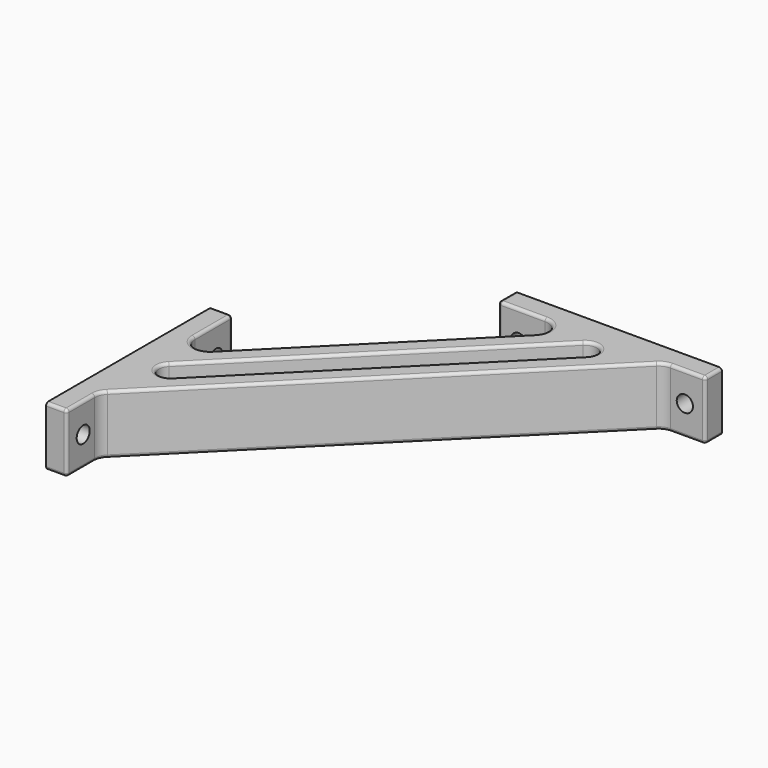
from build123d import *

# Parameters (mm, degrees)
F1_DEPTH       = 20
F6_D           = 5.5
F6_DEPTH       = 7.001
F6_ON_F3_D     = 5.5
F6_ON_F4_D     = 5.5
F6_ON_F4_DEPTH = 7.001
F6_ON_F2_D     = 5.5
F7_R           = 5
F8_R           = 5
F10_DEPTH      = 20.001
F11_R          = 1


# Not quite as in the source:
# - a feature names something its author has since deleted; it is built from what else it names


with BuildPart() as f1:
    # F0 (on Top) → F1 (new body)
    with BuildSketch(Plane.XY):
        Polygon((71.2901826474, 58.548764092), (43.0059113999, 58.548764092), (-34.7758345306, -19.2329818385), (-34.7758345306, -47.517253086), align=None)
        Polygon((85.1480470237, 65.548764092), (15.1480470237, 65.548764092), (15.1480470237, 58.548764092), (43.0059113999, 58.548764092), (71.2901826474, 58.548764092), (85.1480470237, 58.548764092), align=None)
        Polygon((-34.7758345306, -47.517253086), (-34.7758345306, -19.2329818385), (-34.7758345306, 8.6248825378), (-41.7758345306, 8.6248825378), (-41.7758345306, -61.3751174622), (-34.7758345306, -61.3751174622), align=None)
    extrude(amount=-F1_DEPTH)

    # F6 (through all, one way)
    with BuildSketch(Plane.YZ.offset(-34.7758345306)):
        with Locations((1.6958825378, -10)):
            Circle(F6_D / 2)
    extrude(amount=-F6_DEPTH, mode=Mode.SUBTRACT)

    # F6 on F3 (through all)
    with Locations(Plane.YZ.offset(-34.7758345306)):
        with Locations((-54.4461852741, -10)):
            Hole(F6_ON_F3_D / 2)

    # F6 on F4 (through all, one way)
    with BuildSketch(Plane.XZ.offset(-58.548764092)):
        with Locations((22.0770470237, -10)):
            Circle(F6_ON_F4_D / 2)
    extrude(amount=-F6_ON_F4_DEPTH, mode=Mode.SUBTRACT)

    # F6 on F2 (through all)
    with Locations(Plane.XZ.offset(-58.548764092)):
        with Locations((78.2191148355, -10)):
            Hole(F6_ON_F2_D / 2)

    # F7
    f7_edges = [f1.edges().sort_by_distance(p)[0] for p in [
        (-34.775835, -47.517253, -10),
        (71.290183, 58.548764, -10),
    ]]
    fillet(f7_edges, radius=F7_R)

    # F8
    f8_edges = [f1.edges().sort_by_distance(p)[0] for p in [
        (-34.775835, -19.232982, -10),
        (43.005911, 58.548764, -10),
    ]]
    fillet(f8_edges, radius=F8_R)

    # F9 (on face) → F10 (cut, through all)
    with BuildSketch(Plane(origin=(0, 0, -20), x_dir=(1, 0, 0), z_dir=(0, 0, -1))):
        with BuildLine():
            ThreePointArc((47.248552087, -54.3061234049), (52.9054063365, -54.3061234049), (52.9054063365, -48.6492691554))
            Line((52.9054063365, -48.6492691554), (-24.876339594, 29.1324767751))
            ThreePointArc((-24.876339594, 29.1324767751), (-30.5331938435, 29.1324767751), (-30.5331938435, 23.4756225256))
            Line((-30.5331938435, 23.4756225256), (47.248552087, -54.3061234049))
        make_face()
    extrude(amount=-F10_DEPTH, mode=Mode.SUBTRACT)

    # F11
    f11_edges = [f1.edges().sort_by_distance(p)[0] for p in [
        (85.148047, 58.548764, -10),
        (15.148047, 58.548764, -10),
        (-34.775835, 8.624883, -10),
        (-34.775835, -61.375117, -10),
        (14.014533, 9.758396, -20),
        (8.357679, 15.41525, 0),
        (-34.775835, 0.731484, 0),
        (-34.775835, 0.731484, -20),
        (-34.775835, -55.481719, 0),
        (-34.775835, -55.481719, -20),
        (-38.275835, -61.375117, -20),
        (-38.275835, 8.624883, -20),
        (-38.275835, 8.624883, 0),
        (15.148047, 62.048764, -20),
        (85.148047, 62.048764, -20),
        (85.148047, 62.048764, 0),
        (15.148047, 62.048764, 0),
        (-38.275835, -61.375117, 0),
    ]]
    fillet(f11_edges, radius=F11_R)


solid = f1.part
